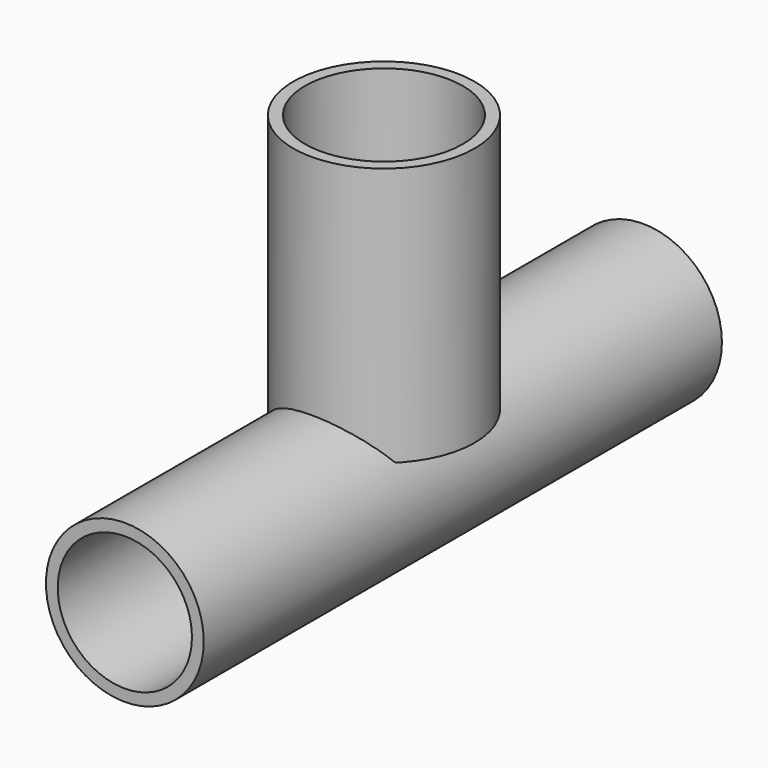
from build123d import *

# Parameters (mm, degrees)
F0_R          = 8.509
F0_R_2        = 7.239
F3_R          = 9.779
F3_R_2        = 8.509
F6_DEPTH      = 20.828
F6_DEPTH_BACK = 5.08
F7_DEPTH      = 5.08


# Not quite as in the source:
# - a feature names something its author has since deleted; it is built from what else it names


with BuildPart() as f2:
    # F2: sweep along a path in F1
    with BuildLine(Plane.YZ) as f2_path:
        Line((0, 0), (-69.85, 0))
    # F0 (on Front) → F2 (sweep)
    with BuildSketch(Plane.XZ):
        Circle(F0_R)
        Circle(F0_R_2, mode=Mode.SUBTRACT)
    sweep(path=f2_path.line)


with BuildPart() as f5:
    # F5: sweep along a path in F4
    with BuildLine(Plane.YZ) as f5_path:
        Line((-34.925, 0), (-34.925, 38.1))
    # F3 (on Top) → F5 (sweep)
    with BuildSketch(Plane.XY):
        with Locations((0, -34.925)):
            Circle(F3_R)
        with Locations((0, -34.925)):
            Circle(F3_R_2, mode=Mode.SUBTRACT)
    sweep(path=f5_path.line)

    # F6 (cut, two sides): a face of the model
    f6_faces = [f5.faces().sort_by_distance(p)[0] for p in [
        (-9.5024081115, -34.925, 0),
    ]]
    extrude(f6_faces, amount=F6_DEPTH, mode=Mode.SUBTRACT)
    extrude(f6_faces, amount=-F6_DEPTH_BACK, mode=Mode.SUBTRACT)

    # F7 (cut): a face of the model
    f7_faces = [f5.faces().sort_by_distance(p)[0] for p in [
        (-9.5024081115, -34.925, 38.1),
    ]]
    extrude(f7_faces, amount=-F7_DEPTH, mode=Mode.SUBTRACT)


solid = Compound([f2.part, f5.part])
